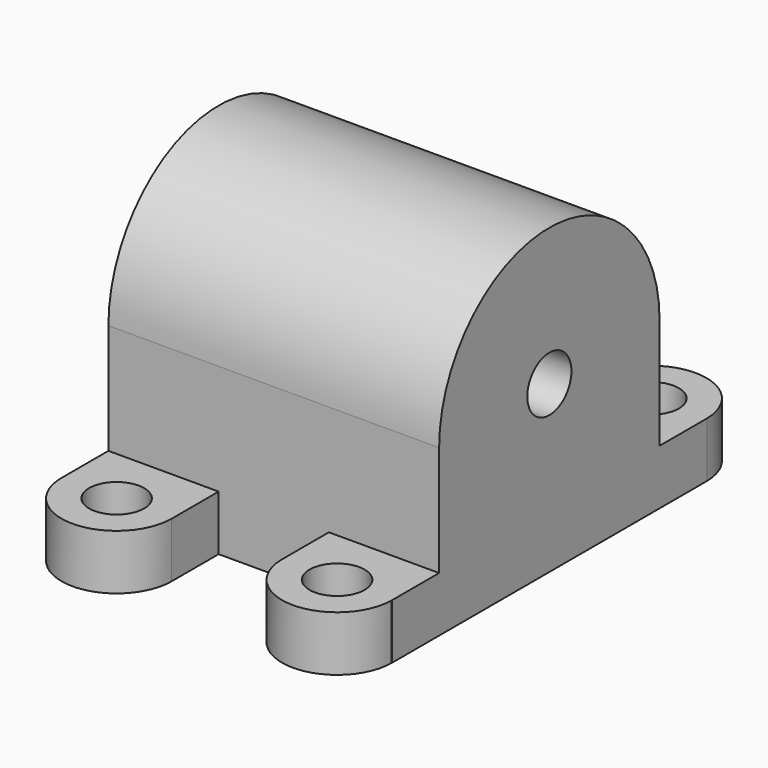
from build123d import *

# Parameters (mm, degrees)
F1_DEPTH = 152.4
F3_R     = 12.7
F4_DEPTH = 25.4
F5_R     = 12.7
F6_DEPTH = 25.4


# Not quite as in the source:
# - a pattern or mirror of a feature is missing from the dataset's text; its kind, count and spacing are read off the source's solid


with BuildPart() as f1:
    # F0 (on Right) → F1 (new body)
    with BuildSketch(Plane.YZ):
        with BuildLine():
            Line((63.5, 12.7), (63.5, 76.2))
            ThreePointArc((63.5, 76.2), (0, 139.7), (-63.5, 76.2))
            Line((-63.5, 76.2), (-63.5, 12.7))
            Line((-63.5, 12.7), (-63.5, 0))
            Line((-63.5, 0), (63.5, 0))
            Line((63.5, 0), (63.5, 12.7))
        make_face()
    extrude(amount=-F1_DEPTH)

    # F3 (on Top) → F4 (join)
    with BuildSketch(Plane.XY):
        with BuildLine():
            Line((0, 90.7872649688), (-0.002730534, 90.7872649688))
            ThreePointArc((-0.002730534, 90.7872649688), (-25.401365267, 115.9239140637), (-50.8, 90.7872649688))
            Line((-50.8, 90.7872649688), (-50.8, 63.5))
            Line((-50.8, 63.5), (0, 63.5))
            Line((0, 63.5), (0, 90.7872649688))
        make_face()
        with Locations((-25.401365267, 90.5239140637)):
            Circle(F3_R, mode=Mode.SUBTRACT)
        with BuildLine():
            Line((-101.6, 90.7872649688), (-101.602730534, 90.7872649688))
            ThreePointArc((-101.602730534, 90.7872649688), (-127.001365267, 115.9239140637), (-152.4, 90.7872649688))
            Line((-152.4, 90.7872649688), (-152.4, 63.5))
            Line((-152.4, 63.5), (-101.6, 63.5))
            Line((-101.6, 63.5), (-101.6, 90.7872649688))
        make_face()
        with Locations((-127.001365267, 90.5239140637)):
            Circle(F3_R, mode=Mode.SUBTRACT)
    f4 = extrude(amount=F4_DEPTH)

    # F4_copies: F4 across plane
    add(f4.mirror(Plane(origin=(0, 0, 0), x_dir=(0, 0, -1), z_dir=(0, -1, 0))))

    # F5 (on face) → F6 (cut)
    with BuildSketch(Plane.YZ):
        with Locations((0, 76.3214752078)):
            Circle(F5_R)
    extrude(amount=-F6_DEPTH, mode=Mode.SUBTRACT)


solid = f1.part
